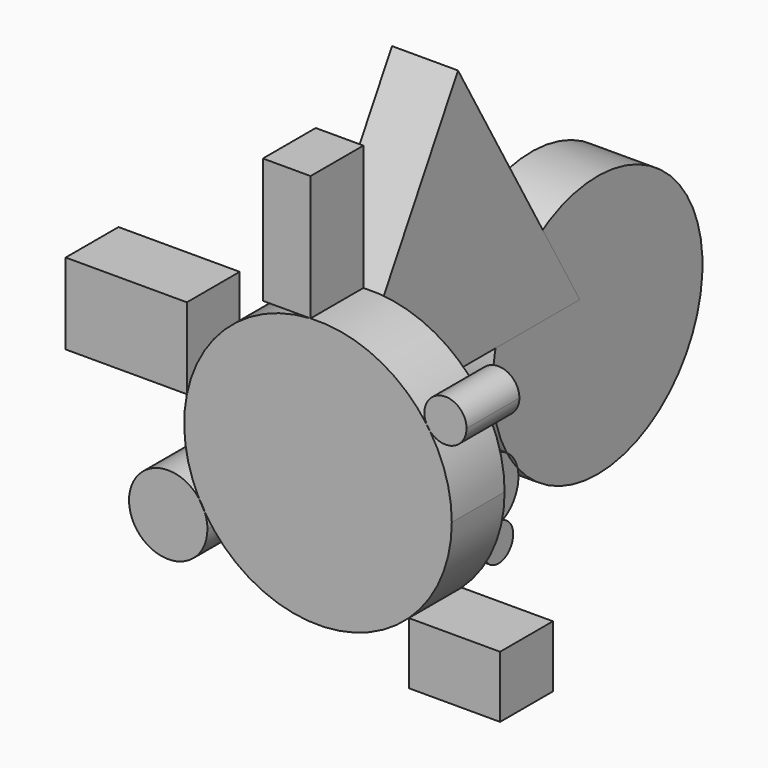
from build123d import *

# Parameters (mm, degrees)
F1_DEPTH = 25.4
F0_W     = 35.1004998692
F0_H     = 23.7618147956
F0_W_2   = 46.6273950725
F0_H_2   = 31.1326426156
F0_W_3   = 18.3327432124
F0_H_3   = 48.2166351118
F3_DEPTH = 25.4
F5_DEPTH = 25.4


with BuildPart() as f1:
    # F0 (on Front) → F1 (new body)
    with BuildSketch(Plane.XZ):
        with BuildLine():
            ThreePointArc((62.9410594702, 42.8905300796), (43.3588603902, 59.2374555897), (18.3327432124, 64.1748591027))
            ThreePointArc((18.3327432124, 64.1748591027), (-12.4706462623, 51.7189218261), (-29.2454881281, 23.0378504209))
            ThreePointArc((-29.2454881281, 23.0378504209), (-29.7872435834, 5.6973312725), (-24.536992326, -10.838144682))
            ThreePointArc((-24.536992326, -10.838144682), (-23.3308600115, -12.63708195), (-22.3948247731, -14.5902251825))
            ThreePointArc((-22.3948247731, -14.5902251825), (14.4291746764, -38.2413882223), (56.1438922278, -25.0025518609))
            ThreePointArc((56.1438922278, -25.0025518609), (68.3541696909, -7.8365718308), (72.6649516178, 12.7832949316))
            ThreePointArc((72.6649516178, 12.7832949316), (70.52758963, 27.4617353398), (64.2930134713, 40.9211182829))
            ThreePointArc((64.2930134713, 40.9211182829), (63.5441553551, 41.855793042), (62.9410594702, 42.8905300796))
        make_face()
    extrude(amount=F1_DEPTH)


with BuildPart() as f1b:
    # F0 (on Front) → F1, piece 2 (new body)
    with BuildSketch(Plane.XZ):
        with Locations((73.6941421624, -36.8834592587)):
            Rectangle(F0_W, F0_H)
    extrude(amount=F1_DEPTH)


with BuildPart() as f1c:
    # F0 (on Front) → F1, piece 3 (new body)
    with BuildSketch(Plane.XZ):
        with Locations((-52.5591856644, 38.6041717287)):
            Rectangle(F0_W_2, F0_H_2)
    extrude(amount=F1_DEPTH)


with BuildPart() as f1d:
    # F0 (on Front) → F1, piece 4 (new body)
    with BuildSketch(Plane.XZ):
        with Locations((9.1663716062, 88.2831766586)):
            Rectangle(F0_W_3, F0_H_3)
    extrude(amount=F1_DEPTH)


with BuildPart() as f1e:
    # F0 (on Front) → F1, piece 5 (new body)
    with BuildSketch(Plane.XZ):
        with BuildLine():
            ThreePointArc((78.3458810146, 46.4474136514), (68.4076058859, 54.3524744917), (62.9410594702, 42.8905300796))
            ThreePointArc((62.9410594702, 42.8905300796), (63.6284631724, 41.9136683381), (64.2930134713, 40.9211182829))
            ThreePointArc((64.2930134713, 40.9211182829), (73.2019635024, 38.8971979808), (78.3458810146, 46.4474136514))
        make_face()
    extrude(amount=F1_DEPTH)


with BuildPart() as f1f:
    # F0 (on Front) → F1, piece 6 (new body)
    with BuildSketch(Plane.XZ):
        with BuildLine():
            ThreePointArc((-22.3948247731, -14.5902251825), (-23.5052950028, -12.7366717585), (-24.536992326, -10.838144682))
            ThreePointArc((-24.536992326, -10.838144682), (-50.6915914862, -25.0203341449), (-21.3464574604, -20.1151670529))
            ThreePointArc((-21.3464574604, -20.1151670529), (-21.6108669498, -17.3034035185), (-22.3948247731, -14.5902251825))
        make_face()
    extrude(amount=F1_DEPTH)


with BuildPart() as f3:
    # F2 (on Right) → F3 (new body)
    with BuildSketch(Plane.YZ):
        with BuildLine():
            ThreePointArc((57.9994903279, -35.7675670337), (63.6084778415, -31.1590847227), (65.7144614914, -24.2118778735))
            ThreePointArc((65.7144614914, -24.2118778735), (65.6155180758, -22.6414926107), (65.3202527329, -21.0959447951))
            ThreePointArc((65.3202527329, -21.0959447951), (62.5671179416, -17.5621102816), (60.1380027846, -13.798184525))
            ThreePointArc((60.1380027846, -13.798184525), (41.3832425563, -20.1080546613), (52.192333573, -36.6827052986))
            ThreePointArc((52.192333573, -36.6827052986), (54.9965455414, -35.5945906676), (57.9994903279, -35.7675670337))
        make_face()
    extrude(amount=F3_DEPTH)


with BuildPart() as f3b:
    # F2 (on Right) → F3, piece 2 (new body)
    with BuildSketch(Plane.YZ):
        with BuildLine():
            ThreePointArc((60.1380027846, -13.798184525), (63.4040352976, -16.9678026085), (65.3202527329, -21.0959447951))
            ThreePointArc((65.3202527329, -21.0959447951), (121.2020574053, -35.7065100131), (154.2361799063, 11.6748308294))
            ThreePointArc((154.2361799063, 11.6748308294), (90.5442953395, 60.4173724355), (60.1380027846, -13.798184525))
        make_face()
    extrude(amount=F3_DEPTH)


with BuildPart() as f3c:
    # F2 (on Right) → F3, piece 3 (new body)
    with BuildSketch(Plane.YZ):
        with BuildLine():
            ThreePointArc((63.1867136248, -42.5951600476), (61.7428184579, -38.307873263), (57.9994903279, -35.7675670337))
            ThreePointArc((57.9994903279, -35.7675670337), (55.1504238642, -36.5710502649), (52.192333573, -36.6827052986))
            ThreePointArc((52.192333573, -36.6827052986), (52.7431673209, -48.8368247671), (63.1867136248, -42.5951600476))
        make_face()
    extrude(amount=F3_DEPTH)


with BuildPart() as f5:
    # F4 (on Right) → F5 (new body)
    with BuildSketch(Plane.YZ):
        Polygon((-21.8691436883, 23.8156784326), (95.2208472725, 23.8156784326), (36.6758517921, 125.2185851336), align=None)
    extrude(amount=F5_DEPTH)


solid = Compound([f1.part, f1b.part, f1c.part, f1d.part, f1e.part, f1f.part, f3.part, f3b.part, f3c.part, f5.part])
